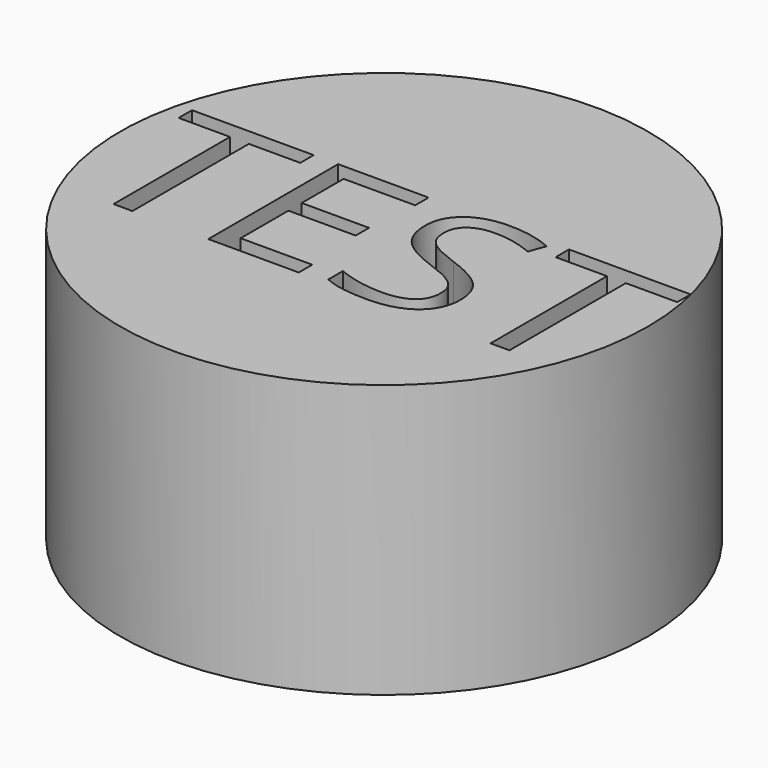
from build123d import *

# Parameters (mm, degrees)
F0_R         = 68.7170921896
F1_DEPTH     = 71.01535
F2_TEXT_SIZE = 59.1786211484
F3_DEPTH     = 20.32298


# Not quite as in the source:
# - Text() gives the source's letters only with a copy of the font that has no kerning and outlines rounded to 1/6400 em; it was checked with that copy


with BuildPart() as f1:
    # F0 (on Top) → F1 (new body)
    with BuildSketch(Plane.XY):
        Circle(F0_R)
    extrude(amount=F1_DEPTH)

    # F2 (on face) → F3 (cut)
    with BuildSketch(Plane.XY.offset(71.01535)):
        with Locations((-63.6975954073, -25.7809056925)):
            Text('TEST', F2_TEXT_SIZE, font='Open Sans', text_align=(TextAlign.LEFT, TextAlign.BOTTOM))
    extrude(amount=-F3_DEPTH, mode=Mode.SUBTRACT)


solid = f1.part
